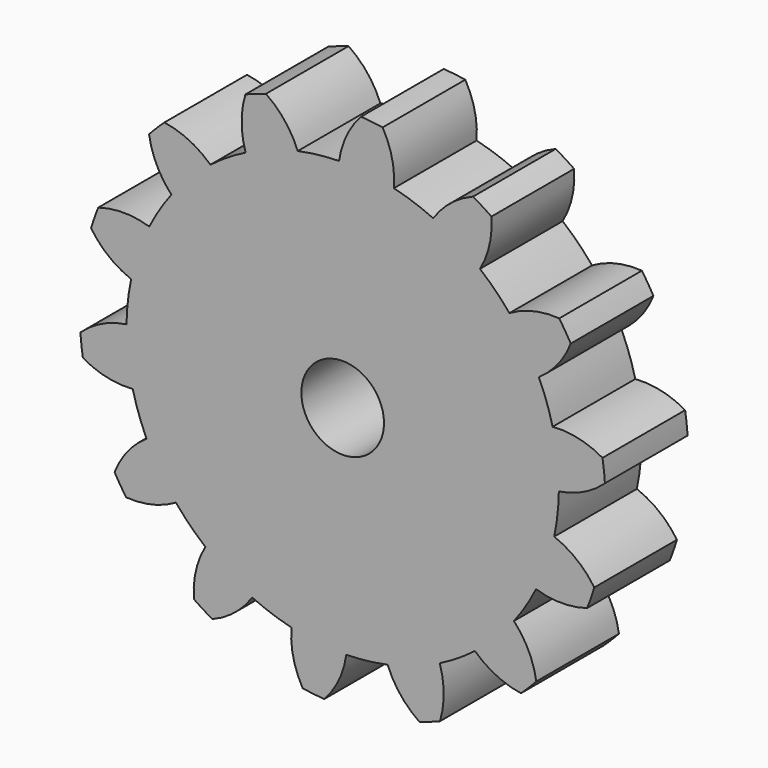
from build123d import *

# Parameters (mm, degrees)
F1_R     = 1.27
F2_DEPTH = 3.175
F3_DEPTH = 3.175
F5_COUNT = 14
F5_ANGLE = 334.2857142857


# Not quite as in the source:
# - a length typed as a fraction of an inch, garbled in the dataset ("3 / 203.2 mm" for 3/8 in), is restored


with BuildPart() as f2:
    # F1 (on Front) → F2 (new body)
    with BuildSketch(Plane.XZ):
        with BuildLine():
            ThreePointArc((6.6428889328, -0.0990154985), (6.6434423524, -0.049509124), (6.643626829, 0))
            ThreePointArc((6.643626829, 0), (6.5953592641, 0.7993832744), (6.4512579209, 1.587151121))
            ThreePointArc((6.4512579209, 1.587151121), (-6.6011332303, -0.7502116494), (6.6428889328, -0.0990154985))
        make_face()
        Circle(F1_R, mode=Mode.SUBTRACT)
    extrude(amount=F2_DEPTH)

    # F1 (on Front) → F3 (join)
    with BuildSketch(Plane.XZ):
        with BuildLine():
            ThreePointArc((6.4512579209, 1.587151121), (6.5953592641, 0.7993832744), (6.643626829, 0))
            ThreePointArc((6.643626829, 0), (6.6434423524, -0.049509124), (6.6428889328, -0.0990154985))
            ThreePointArc((6.6428889328, -0.0990154985), (7.4027472944, 0.1325210174), (8.0591667411, 0.5798546712))
            ThreePointArc((8.0591667411, 0.5798546712), (8.0283191506, 0.9124097851), (7.9837548494, 1.2434060096))
            ThreePointArc((7.9837548494, 1.2434060096), (7.2436944715, 1.5320312423), (6.4512579209, 1.587151121))
        make_face()
    extrude(amount=F3_DEPTH)

    # F5: F2 ×14 about axis
    f5_axis = Axis((0, 6.1465417966, 0), (0, 1, 0))


with BuildPart() as f2_1:
    add(f2.part)
    for i in range(1, F5_COUNT):
        add(f2.part.rotate(f5_axis, i * F5_ANGLE / (F5_COUNT - 1)))


solid = f2_1.part
